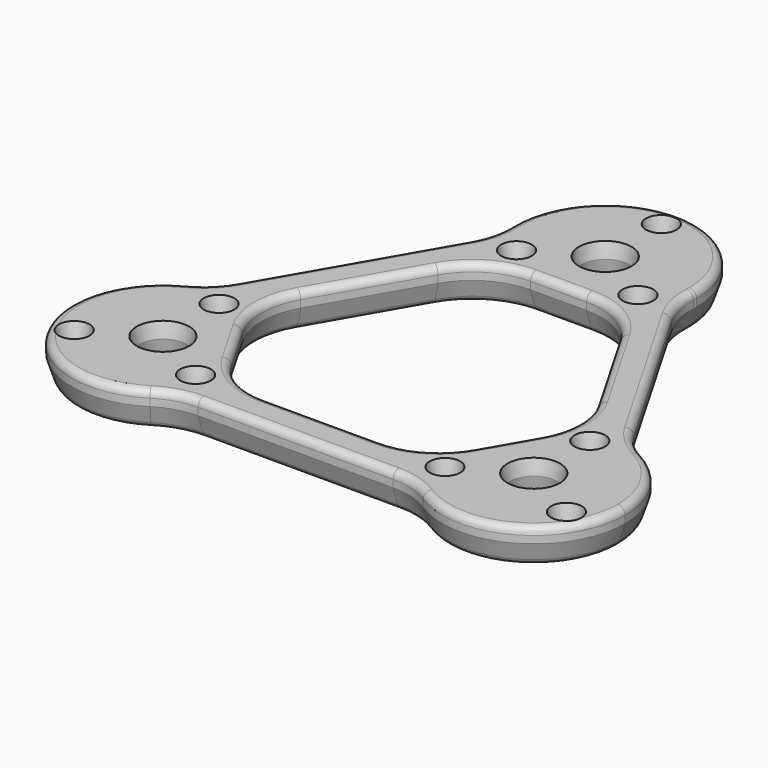
from build123d import *

# Parameters (mm, degrees)
F0_R     = 1.7
F0_R_2   = 3.2
F1_DEPTH = 5
F2_DEPTH = 0.4
F3_SIZE2 = 3
F3_SIZE  = 0.6
F4_R     = 10
F5_SIZE2 = 3
F5_SIZE  = 1
F6_R     = 1
F8_R     = 1
F9_SIZE  = 0.6


# Not quite as in the source:
# - a fillet or chamfer that OpenCascade refuses, or shapes differently, is made with other operations: its cross-section is extruded or revolved along the edge and cut away or added


with BuildPart() as f1:
    # F0 (on Top) → F1 (new body)
    with BuildSketch(Plane.XY):
        with BuildLine():
            ThreePointArc((12.1346610995, 26.4457274827), (12.408329133, 27.9346457086), (12.5, 29.4457274827))
            ThreePointArc((12.5, 29.4457274827), (-1.5110817741, 41.8540566156), (-12.1346610995, 26.4457274827))
            ThreePointArc((-12.1346610995, 26.4457274827), (-11.1534661406, 23.8021299553), (-9.6046863561, 21.4457274827))
            Line((-9.6046863561, 21.4457274827), (9.6046863561, 21.4457274827))
            ThreePointArc((9.6046863561, 21.4457274827), (11.1534661406, 23.8021299553), (12.1346610995, 26.4457274827))
        make_face()
        with Locations((-8.3138438763, 24.6457274827)):
            Circle(F0_R, mode=Mode.SUBTRACT)
        with Locations((8.3138438763, 24.6457274827)):
            Circle(F0_R, mode=Mode.SUBTRACT)
        with Locations((0, 29.4457274827)):
            Circle(F0_R_2, mode=Mode.SUBTRACT)
        with Locations((0, 39.0457274827)):
            Circle(F0_R, mode=Mode.SUBTRACT)
        with BuildLine():
            ThreePointArc((-9.6046863561, 21.4457274827), (-11.1534661406, 23.8021299553), (-12.1346610995, 26.4457274827))
            Line((-12.1346610995, 26.4457274827), (-28.859740605, -2.5229599815))
            ThreePointArc((-28.859740605, -2.5229599815), (-26.0797205095, -2.0509009783), (-23.2646262144, -2.2139823802))
            Line((-23.2646262144, -2.2139823802), (-9.6046863561, 21.4457274827))
        make_face()
        with BuildLine():
            Line((28.859740605, -2.5229599815), (12.1346610995, 26.4457274827))
            ThreePointArc((12.1346610995, 26.4457274827), (11.1534661406, 23.8021299553), (9.6046863561, 21.4457274827))
            Line((9.6046863561, 21.4457274827), (23.2646262144, -2.2139823802))
            ThreePointArc((23.2646262144, -2.2139823802), (26.0797205095, -2.0509009783), (28.859740605, -2.5229599815))
        make_face()
        with BuildLine():
            ThreePointArc((-23.2646262144, -2.2139823802), (-26.0797205095, -2.0509009783), (-28.859740605, -2.5229599815))
            ThreePointArc((-28.859740605, -2.5229599815), (-36.2158038139, -20.78188476), (-16.7250795055, -23.5408095385))
            ThreePointArc((-16.7250795055, -23.5408095385), (-14.9262543689, -21.3692710143), (-13.6599398583, -18.8497871398))
            Line((-13.6599398583, -18.8497871398), (-23.2646262144, -2.2139823802))
        make_face()
        with Locations((-33.704330143, -19.33188476)):
            Circle(F0_R, mode=Mode.SUBTRACT)
        with Locations((-25.3904862666, -14.53188476)):
            Circle(F0_R_2, mode=Mode.SUBTRACT)
        with Locations((-17.0766423903, -19.33188476)):
            Circle(F0_R, mode=Mode.SUBTRACT)
        with Locations((-25.3904862666, -4.93188476)):
            Circle(F0_R, mode=Mode.SUBTRACT)
        with BuildLine():
            ThreePointArc((37.8904862666, -14.53188476), (35.3808736272, -7.0190849899), (28.859740605, -2.5229599815))
            ThreePointArc((28.859740605, -2.5229599815), (26.0797205095, -2.0509009783), (23.2646262144, -2.2139823802))
            Line((23.2646262144, -2.2139823802), (13.6599398583, -18.8497871398))
            ThreePointArc((13.6599398583, -18.8497871398), (14.9262543689, -21.3692710143), (16.7250795055, -23.5408095385))
            ThreePointArc((16.7250795055, -23.5408095385), (30.2860156295, -26.0333538947), (37.8904862666, -14.53188476))
        make_face()
        with Locations((17.0766423903, -19.33188476)):
            Circle(F0_R, mode=Mode.SUBTRACT)
        with Locations((33.704330143, -19.33188476)):
            Circle(F0_R, mode=Mode.SUBTRACT)
        with Locations((25.3904862666, -14.53188476)):
            Circle(F0_R_2, mode=Mode.SUBTRACT)
        with Locations((25.3904862666, -4.93188476)):
            Circle(F0_R, mode=Mode.SUBTRACT)
        with BuildLine():
            ThreePointArc((-13.6599398583, -18.8497871398), (-14.9262543689, -21.3692710143), (-16.7250795055, -23.5408095385))
            Line((-16.7250795055, -23.5408095385), (16.7250795055, -23.5408095385))
            ThreePointArc((16.7250795055, -23.5408095385), (14.9262543689, -21.3692710143), (13.6599398583, -18.8497871398))
            Line((13.6599398583, -18.8497871398), (-13.6599398583, -18.8497871398))
        make_face()
    extrude(amount=F1_DEPTH)

    # F0 (on Top) → F2 (join)
    with BuildSketch(Plane.XY):
        with Locations((33.704330143, -19.33188476)):
            Circle(F0_R)
        with Locations((25.3904862666, -4.93188476)):
            Circle(F0_R)
        with Locations((0, 39.0457274827)):
            Circle(F0_R)
        with Locations((-25.3904862666, -4.93188476)):
            Circle(F0_R)
        with Locations((-17.0766423903, -19.33188476)):
            Circle(F0_R)
        with Locations((-33.704330143, -19.33188476)):
            Circle(F0_R)
        with Locations((17.0766423903, -19.33188476)):
            Circle(F0_R)
        with Locations((8.3138438763, 24.6457274827)):
            Circle(F0_R)
        with Locations((-8.3138438763, 24.6457274827)):
            Circle(F0_R)
    extrude(amount=F2_DEPTH)

    # F3
    f3_edges = [f1.edges().sort_by_distance(p)[0] for p in [
        (-28.590486, -14.531885, 0),
        (22.190486, -14.531885, 0),
        (-3.2, 29.445727, 0),
    ]]
    f3_side = f1.faces().sort_by_distance((0, 40.921, 0))[0]
    chamfer(f3_edges, length=F3_SIZE, length2=F3_SIZE2, reference=f3_side)

    # F4
    f4_edges = [f1.edges().sort_by_distance(p)[0] for p in [
        (-9.604686, 21.445727, 2.5),
        (9.604686, 21.445727, 2.5),
        (-23.264626, -2.213982, 2.5),
        (-13.65994, -18.849787, 2.5),
        (13.65994, -18.849787, 2.5),
        (23.264626, -2.213982, 2.5),
        (16.72508, -23.54081, 2.5),
        (-16.72508, -23.54081, 2.5),
        (-28.859741, -2.52296, 2.5),
        (-12.134661, 26.445727, 2.5),
        (12.134661, 26.445727, 2.5),
        (28.859741, -2.52296, 2.5),
    ]]
    fillet(f4_edges, radius=F4_R)

    # F5
    f5_edges = [f1.edges().sort_by_distance(p)[0] for p in [
        (20.497201, 11.961384, 0),
        (16.434656, 9.615873, 0),
    ]]
    f5_side = f1.faces().sort_by_distance((0, 40.921, 0))[0]
    chamfer(f5_edges, length=F5_SIZE, length2=F5_SIZE2, reference=f5_side)

    # F6
    f6_edges = [f1.edges().sort_by_distance(p)[0] for p in [
        (0, -18.849787, 5),
        (20.497201, 11.961384, 5),
    ]]
    fillet(f6_edges, radius=F6_R)

    # F7: chamfer of 0.4 x 2 on 12 edges, made by hand

    # F7_s1 → F7_t2 (revolve, cut)
    with BuildSketch(Plane.XZ.offset(4.93188476)):
        Polygon((27.4904862666, 5), (27.0904862666, 3), (27.0904862666, 5), align=None)
    revolve(axis=Axis((25.3904862666, -4.93188476, 5), (0, 0, 1)), mode=Mode.SUBTRACT)

    # F7_s3 → F7_t4 (revolve, cut)
    with BuildSketch(Plane.XZ.offset(19.33188476)):
        Polygon((19.1766423903, 5), (18.7766423903, 3), (18.7766423903, 5), align=None)
    revolve(axis=Axis((17.0766423903, -19.33188476, 5), (0, 0, 1)), mode=Mode.SUBTRACT)

    # F7_s5 → F7_t6 (revolve, cut)
    with BuildSketch(Plane.XZ.offset(19.33188476)):
        Polygon((35.804330143, 5), (35.404330143, 3), (35.404330143, 5), align=None)
    revolve(axis=Axis((33.704330143, -19.33188476, 5), (0, 0, 1)), mode=Mode.SUBTRACT)

    # F7_s7 → F7_t8 (revolve, cut)
    with BuildSketch(Plane.XZ.offset(19.33188476)):
        Polygon((-31.604330143, 5), (-32.004330143, 3), (-32.004330143, 5), align=None)
    revolve(axis=Axis((-33.704330143, -19.33188476, 5), (0, 0, 1)), mode=Mode.SUBTRACT)

    # F7_s9 → F7_t10 (revolve, cut)
    with BuildSketch(Plane.XZ.offset(19.33188476)):
        Polygon((-14.9766423903, 5), (-15.3766423903, 3), (-15.3766423903, 5), align=None)
    revolve(axis=Axis((-17.0766423903, -19.33188476, 5), (0, 0, 1)), mode=Mode.SUBTRACT)

    # F7_s11 → F7_t12 (revolve, cut)
    with BuildSketch(Plane.XZ.offset(4.93188476)):
        Polygon((-23.2904862666, 5), (-23.6904862666, 3), (-23.6904862666, 5), align=None)
    revolve(axis=Axis((-25.3904862666, -4.93188476, 5), (0, 0, 1)), mode=Mode.SUBTRACT)

    # F7_s13 → F7_t14 (revolve, cut)
    with BuildSketch(Plane.XZ.offset(-24.6457274827)):
        Polygon((10.4138438763, 5), (10.0138438763, 3), (10.0138438763, 5), align=None)
    revolve(axis=Axis((8.3138438763, 24.6457274827, 5), (0, 0, 1)), mode=Mode.SUBTRACT)

    # F7_s15 → F7_t16 (revolve, cut)
    with BuildSketch(Plane.XZ.offset(-24.6457274827)):
        Polygon((-6.2138438763, 5), (-6.6138438763, 3), (-6.6138438763, 5), align=None)
    revolve(axis=Axis((-8.3138438763, 24.6457274827, 5), (0, 0, 1)), mode=Mode.SUBTRACT)

    # F7_s17 → F7_t18 (revolve, cut)
    with BuildSketch(Plane.XZ.offset(-39.0457274827)):
        Polygon((2.1, 5), (1.7, 3), (1.7, 5), align=None)
    revolve(axis=Axis((0, 39.0457274827, 5), (0, 0, 1)), mode=Mode.SUBTRACT)

    # F7_s19 → F7_t20 (revolve, cut)
    with BuildSketch(Plane.XZ.offset(14.53188476)):
        Polygon((28.9904862666, 5), (28.5904862666, 3), (28.5904862666, 5), align=None)
    revolve(axis=Axis((25.3904862666, -14.53188476, 5), (0, 0, 1)), mode=Mode.SUBTRACT)

    # F7_s21 → F7_t22 (revolve, cut)
    with BuildSketch(Plane.XZ.offset(-29.4457274827)):
        Polygon((3.6, 5), (3.2, 3), (3.2, 5), align=None)
    revolve(axis=Axis((0, 29.4457274827, 5), (0, 0, 1)), mode=Mode.SUBTRACT)

    # F7_s23 → F7_t24 (revolve, cut)
    with BuildSketch(Plane.XZ.offset(14.53188476)):
        Polygon((-21.7904862666, 5), (-22.1904862666, 3), (-22.1904862666, 5), align=None)
    revolve(axis=Axis((-25.3904862666, -14.53188476, 5), (0, 0, 1)), mode=Mode.SUBTRACT)

    # F8
    f8_edges = [f1.edges().sort_by_distance(p)[0] for p in [
        (0, -22.54081, 0),
        (0, -19.849787, 0),
        (19.631175, 11.461384, 0),
        (28.216375, -2.538017, 0),
        (11.799938, 25.896085, 0),
        (35.349778, -20.281885, 0),
        (0, 40.945727, 0),
        (16.416437, -22.97611, 0),
        (-11.799938, 25.896085, 0),
        (-19.631175, 11.461384, 0),
        (-16.416437, -22.97611, 0),
        (-28.216375, -2.538017, 0),
        (-35.349778, -20.281885, 0),
        (17.300682, 10.115873, 0),
        (9.331184, 20.972007, 0),
        (22.717621, -2.213982, 0),
        (0, 22.445727, 0),
        (19.328308, -11.031885, 0),
        (-9.331184, 20.972007, 0),
        (13.386437, -18.376067, 0),
        (-17.300682, 10.115873, 0),
        (-22.717621, -2.213982, 0),
        (-13.386437, -18.376067, 0),
        (-19.328308, -11.031885, 0),
    ]]
    fillet(f8_edges, radius=F8_R)

    # F9
    f9_edges = [f1.edges().sort_by_distance(p)[0] for p in [
        (-18.776642, -19.331885, 0.4),
        (-27.090486, -4.931885, 0.4),
        (-35.40433, -19.331885, 0.4),
        (32.00433, -19.331885, 0.4),
        (15.376642, -19.331885, 0.4),
        (23.690486, -4.931885, 0.4),
        (6.613844, 24.645727, 0.4),
        (-10.013844, 24.645727, 0.4),
        (-1.7, 39.045727, 0.4),
    ]]
    chamfer(f9_edges, length=F9_SIZE)


solid = f1.part
